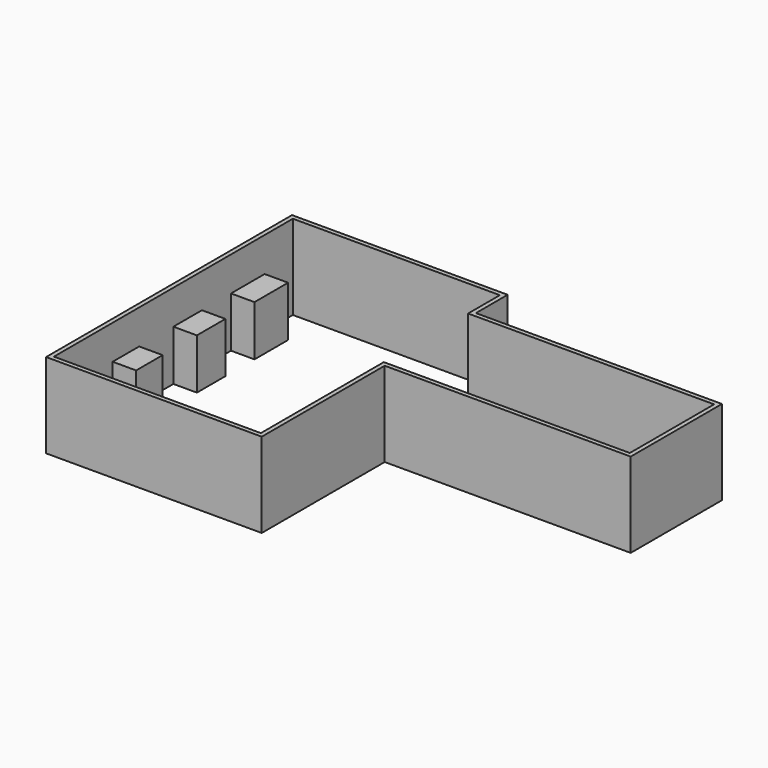
from build123d import *

# Parameters (mm, degrees)
F0_W     = 143.7272205949
F0_H     = 66.6242633015
F1_DEPTH = 49.53
F2_T     = -2.54
F3_W     = 13.7264372474
F3_H     = 19.3594098091
F3_H_2   = 20.8327490836
F3_H_3   = 24.5586633682
F4_DEPTH = 29.464


with BuildPart() as f1:
    # F0 (on Top) → F1 (new body)
    with BuildSketch(Plane.XY):
        Polygon((-16.2664372474, 189.0449970961), (-16.2664372474, 9.442742914), (109.7329184413, 9.442742914), (109.7329184413, 99.243870005), (109.7329184413, 165.8681333065), (109.7329184413, 189.0449970961), align=None)
        with Locations((181.5965287387, 132.5560016558)):
            Rectangle(F0_W, F0_H)
    extrude(amount=F1_DEPTH)

    # F2
    f2_openings = [f1.faces().sort_by_distance(p)[0] for p in [
        (86.832403, 109.148631, 49.53),
        (86.832403, 109.148631, 0),
    ]]
    offset(amount=F2_T, openings=f2_openings, kind=Kind.INTERSECTION)

    # F3 (on Top) → F4 (join)
    with BuildSketch(Plane.XY):
        with Locations((-6.8632186237, 64.5605772734)):
            Rectangle(F3_W, F3_H)
        with Locations((-6.8632186237, 109.6602445468)):
            Rectangle(F3_W, F3_H_2)
        with Locations((-6.8632186237, 153.5996198654)):
            Rectangle(F3_W, F3_H_3)
    extrude(amount=F4_DEPTH)


solid = f1.part
